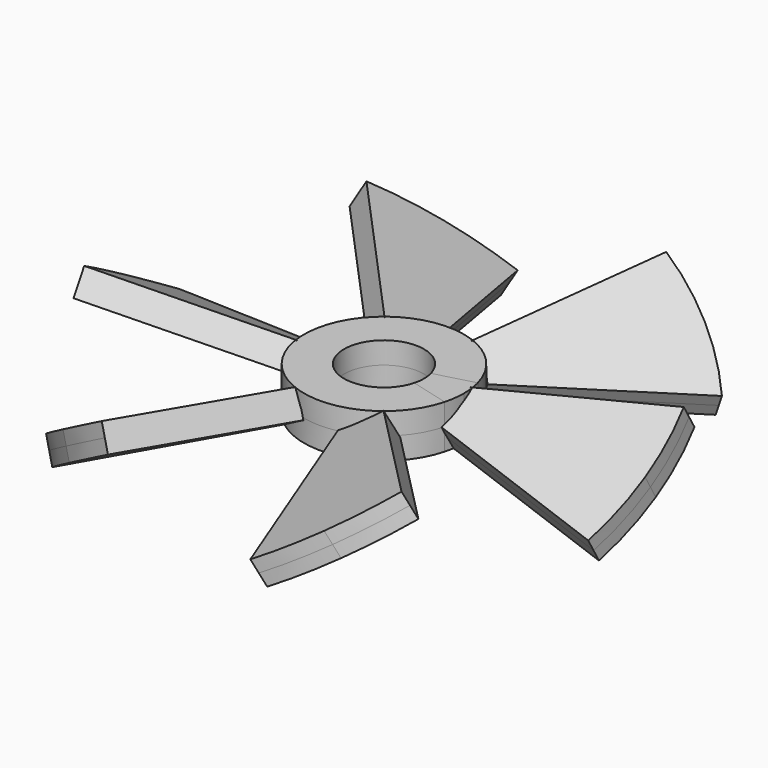
from build123d import *

# Parameters (mm, degrees)
F1_DEPTH      = 5
F1_DEPTH_BACK = 5
F2_ANGLE      = 30
F4_COUNT      = 6
F5_DEPTH      = 8.2124126955
F6_DEPTH      = 8.2124126955
F7_DEPTH      = 8.2124126955


with BuildPart() as f1:
    # F0 (on Top) → F1 (new body, two sides)
    with BuildSketch(Plane.XY) as f1_sk:
        with BuildLine():
            ThreePointArc((28.9777747887, 7.7645713531), (29.7433458412, 3.9157857666), (30, 0))
            Line((30, 0), (100, 0))
            ThreePointArc((100, 0), (99.1444861374, 13.052619222), (96.5925826289, 25.8819045103))
            Line((96.5925826289, 25.8819045103), (28.9777747887, 7.7645713531))
        make_face()
        with BuildLine():
            Line((100, 0), (30, 0))
            ThreePointArc((30, 0), (29.7433458412, -3.9157857666), (28.9777747887, -7.7645713531))
            Line((28.9777747887, -7.7645713531), (96.5925826289, -25.8819045103))
            ThreePointArc((96.5925826289, -25.8819045103), (99.1444861374, -13.052619222), (100, 0))
        make_face()
    extrude(amount=F1_DEPTH)
    extrude(f1_sk.sketch, amount=-F1_DEPTH_BACK)


with BuildPart() as f1_1:
    # F2: moved
    add(f1.part.rotate(Axis((50, 0, 0), (1, 0, 0)), F2_ANGLE))


with BuildPart() as f4_1:
    # F4: instance of F1
    add(f1_1.part.rotate(Axis((0, 0, 27.5022108108), (0, 0, 1)), 1 * 360 / F4_COUNT))


with BuildPart() as f4_2:
    # F4: instance of F1
    add(f1_1.part.rotate(Axis((0, 0, 27.5022108108), (0, 0, 1)), 2 * 360 / F4_COUNT))


with BuildPart() as f4_3:
    # F4: instance of F1
    add(f1_1.part.rotate(Axis((0, 0, 27.5022108108), (0, 0, 1)), 3 * 360 / F4_COUNT))


with BuildPart() as f4_4:
    # F4: instance of F1
    add(f1_1.part.rotate(Axis((0, 0, 27.5022108108), (0, 0, 1)), 4 * 360 / F4_COUNT))


with BuildPart() as f4_5:
    # F4: instance of F1
    add(f1_1.part.rotate(Axis((0, 0, 27.5022108108), (0, 0, 1)), 5 * 360 / F4_COUNT))


with BuildPart() as f5:
    # F0 (on Top) → F5 (new body, through all)
    with BuildSketch(Plane.XY):
        with BuildLine():
            ThreePointArc((14.4888873943, -3.8822856765), (-15, 0), (14.4888873943, 3.8822856765))
            Line((14.4888873943, 3.8822856765), (28.9777747887, 7.7645713531))
            ThreePointArc((28.9777747887, 7.7645713531), (-30, 0), (28.9777747887, -7.7645713531))
            Line((28.9777747887, -7.7645713531), (14.4888873943, -3.8822856765))
        make_face()
    extrude(amount=F5_DEPTH)


with BuildPart() as f6:
    # F0 (on Top) → F6 (new body, through all)
    with BuildSketch(Plane.XY):
        with BuildLine():
            ThreePointArc((14.4888873943, 3.8822856765), (14.8716729206, 1.9578928833), (15, 0))
            Line((15, 0), (30, 0))
            ThreePointArc((30, 0), (29.7433458412, 3.9157857666), (28.9777747887, 7.7645713531))
            Line((28.9777747887, 7.7645713531), (14.4888873943, 3.8822856765))
        make_face()
        with BuildLine():
            Line((30, 0), (15, 0))
            ThreePointArc((15, 0), (14.8716729206, -1.9578928833), (14.4888873943, -3.8822856765))
            Line((14.4888873943, -3.8822856765), (28.9777747887, -7.7645713531))
            ThreePointArc((28.9777747887, -7.7645713531), (29.7433458412, -3.9157857666), (30, 0))
        make_face()
    extrude(amount=F6_DEPTH)


with BuildPart() as f7:
    # F0 (on Top) → F7 (new body, through all)
    with BuildSketch(Plane.XY):
        with BuildLine():
            ThreePointArc((14.4888873943, -3.8822856765), (-15, 0), (14.4888873943, 3.8822856765))
            Line((14.4888873943, 3.8822856765), (28.9777747887, 7.7645713531))
            ThreePointArc((28.9777747887, 7.7645713531), (-30, 0), (28.9777747887, -7.7645713531))
            Line((28.9777747887, -7.7645713531), (14.4888873943, -3.8822856765))
        make_face()
        with BuildLine():
            Line((30, 0), (15, 0))
            ThreePointArc((15, 0), (14.8716729206, -1.9578928833), (14.4888873943, -3.8822856765))
            Line((14.4888873943, -3.8822856765), (28.9777747887, -7.7645713531))
            ThreePointArc((28.9777747887, -7.7645713531), (29.7433458412, -3.9157857666), (30, 0))
        make_face()
        with BuildLine():
            ThreePointArc((14.4888873943, 3.8822856765), (14.8716729206, 1.9578928833), (15, 0))
            Line((15, 0), (30, 0))
            ThreePointArc((30, 0), (29.7433458412, 3.9157857666), (28.9777747887, 7.7645713531))
            Line((28.9777747887, 7.7645713531), (14.4888873943, 3.8822856765))
        make_face()
    extrude(amount=-F7_DEPTH)


solid = Compound([f1_1.part, f4_1.part, f4_2.part, f4_3.part, f4_4.part, f4_5.part, f5.part, f6.part, f7.part])
